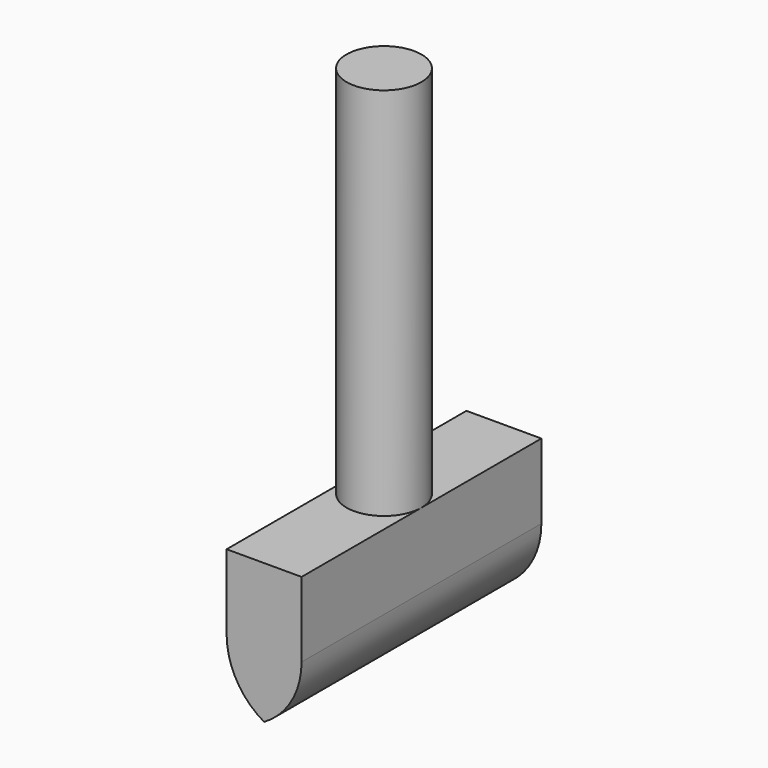
from build123d import *

# Parameters (mm, degrees)
F0_W        = 5
F0_H        = 10
F1_DEPTH    = 20
F2_T1_DEPTH = 45
F3_R        = 2.5
F4_DEPTH    = 25


# Not quite as in the source:
# - a fillet or chamfer that OpenCascade refuses, or shapes differently, is made with other operations: its cross-section is extruded or revolved along the edge and cut away or added


with BuildPart() as f1:
    # F0 (on Front) → F1 (new body)
    with BuildSketch(Plane.XZ):
        Rectangle(F0_W, F0_H)
    extrude(amount=F1_DEPTH)

    # F2: fillet of radius 5 on 2 edges, made by hand

    # F2_s2 → F2_t1 (cut)
    with BuildSketch(Plane.XZ.offset(-12.5)):
        with BuildLine():
            ThreePointArc((-2.5, 0), (-1.0355339059, -3.5355339059), (2.5, -5))
            Line((2.5, -5), (-2.5, -5))
            Line((-2.5, -5), (-2.5, 0))
        make_face()
        with BuildLine():
            ThreePointArc((-2.5, -5), (1.0355339059, -3.5355339059), (2.5, 0))
            Line((2.5, 0), (2.5, -5))
            Line((2.5, -5), (-2.5, -5))
        make_face()
    extrude(amount=F2_T1_DEPTH, mode=Mode.SUBTRACT)

    # F3 (on face) → F4 (join)
    with BuildSketch(Plane.XY.offset(5)):
        with Locations((0, -10)):
            Circle(F3_R)
    extrude(amount=F4_DEPTH)


solid = f1.part
